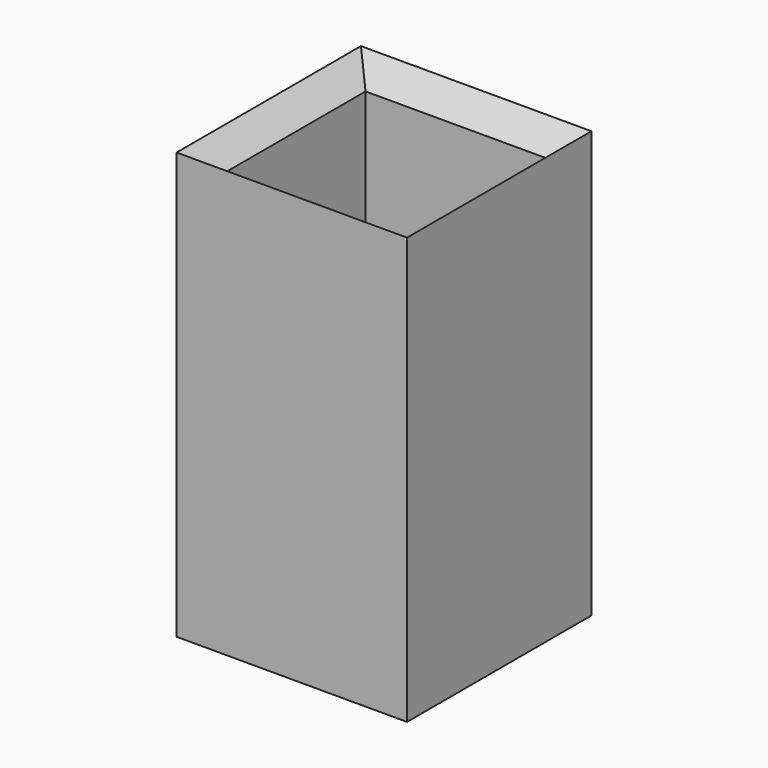
from build123d import *

# Parameters (mm, degrees)
F0_W         = 25.4
F0_H         = 25.4
F0_W_2       = 20.32
F0_H_2       = 20.32
F1_DEPTH     = 50.8
F2_T1_DEPTH  = 20.32
F2_T3_DEPTH  = 20.32
F2_T9_DEPTH  = 36.6501869736
F2_T15_DEPTH = 36.6501869736
F2_T24_DEPTH = 36.6501869736
F2_T30_DEPTH = 36.6501869736
F2_T39_DEPTH = 36.6501869736
F2_T45_DEPTH = 36.6501869736
F2_T54_DEPTH = 36.6501869736
F2_T60_DEPTH = 36.6501869736


# Not quite as in the source:
# - a fillet or chamfer that OpenCascade refuses, or shapes differently, is made with other operations: its cross-section is extruded or revolved along the edge and cut away or added


with BuildPart() as f1:
    # F0 (on Top) → F1 (new body)
    with BuildSketch(Plane.XY):
        Rectangle(F0_W, F0_H)
        Rectangle(F0_W_2, F0_H_2, mode=Mode.SUBTRACT)
    extrude(amount=F1_DEPTH)

    # F2: chamfer of 6.35 on 4 edges, made by hand

    # F2_s2 → F2_t1 (cut)
    with BuildSketch(Plane.XZ.offset(-10.16)):
        Polygon((-10.16, 44.45), (-16.51, 50.8), (-10.16, 50.8), align=None)
        Polygon((10.16, 44.45), (16.51, 50.8), (10.16, 50.8), align=None)
    extrude(amount=F2_T1_DEPTH, mode=Mode.SUBTRACT)

    # F2_s4 → F2_t3 (cut)
    with BuildSketch(Plane.YZ.offset(-10.16)):
        Polygon((-10.16, 44.45), (-16.51, 50.8), (-10.16, 50.8), align=None)
        Polygon((10.16, 44.45), (16.51, 50.8), (10.16, 50.8), align=None)
    extrude(amount=F2_T3_DEPTH, mode=Mode.SUBTRACT)


with BuildPart() as f2_tool7:
    # F2_s8 → F2_t9 (new body)
    with BuildSketch(Plane.YZ.offset(10.16)):
        Polygon((-10.16, 44.45), (-16.51, 50.8), (-10.16, 50.8), align=None)
    extrude(amount=-F2_T9_DEPTH)

    split(bisect_by=Plane.XZ.offset(12.7), keep=Keep.BOTTOM)

    split(bisect_by=Plane.YZ.offset(-12.7), keep=Keep.TOP)

    split(bisect_by=Plane.YZ.offset(-10.16), keep=Keep.BOTTOM)


with BuildPart() as f2_tool13:
    # F2_s14 → F2_t15 (new body)
    with BuildSketch(Plane.XZ.offset(26.4901869736)):
        Polygon((-10.16, 44.45), (-16.51, 50.8), (-10.16, 50.8), align=None)
    extrude(amount=-F2_T15_DEPTH)

    split(bisect_by=Plane.XZ.offset(12.7), keep=Keep.BOTTOM)

    split(bisect_by=Plane.YZ.offset(-12.7), keep=Keep.TOP)

    split(bisect_by=Plane.XZ.offset(10.16), keep=Keep.TOP)


with BuildPart() as f2_tool7_1:
    add(f2_tool7.part)

    # F2_t19: intersect F2_tool13
    add(f2_tool13.part, mode=Mode.INTERSECT)


with BuildPart() as f1_1:
    add(f1.part)

    # F2_t5: cut F2_tool7
    add(f2_tool7_1.part, mode=Mode.SUBTRACT)


with BuildPart() as f2_tool22:
    # F2_s23 → F2_t24 (new body)
    with BuildSketch(Plane.YZ.offset(-26.4901869736)):
        Polygon((10.16, 44.45), (16.51, 50.8), (10.16, 50.8), align=None)
    extrude(amount=F2_T24_DEPTH)

    split(bisect_by=Plane.XZ.offset(-12.7), keep=Keep.TOP)

    split(bisect_by=Plane.YZ.offset(-12.7), keep=Keep.TOP)

    split(bisect_by=Plane.YZ.offset(-10.16), keep=Keep.BOTTOM)


with BuildPart() as f2_tool28:
    # F2_s29 → F2_t30 (new body)
    with BuildSketch(Plane.XZ.offset(10.16)):
        Polygon((-10.16, 44.45), (-16.51, 50.8), (-10.16, 50.8), align=None)
    extrude(amount=-F2_T30_DEPTH)

    split(bisect_by=Plane.XZ.offset(-12.7), keep=Keep.TOP)

    split(bisect_by=Plane.YZ.offset(-12.7), keep=Keep.TOP)

    split(bisect_by=Plane.XZ.offset(-10.16), keep=Keep.BOTTOM)


with BuildPart() as f2_tool22_1:
    add(f2_tool22.part)

    # F2_t34: intersect F2_tool28
    add(f2_tool28.part, mode=Mode.INTERSECT)


with BuildPart() as f1_2:
    add(f1_1.part)

    # F2_t20: cut F2_tool22
    add(f2_tool22_1.part, mode=Mode.SUBTRACT)


with BuildPart() as f2_tool37:
    # F2_s38 → F2_t39 (new body)
    with BuildSketch(Plane.YZ.offset(-10.16)):
        Polygon((10.16, 44.45), (16.51, 50.8), (10.16, 50.8), align=None)
    extrude(amount=F2_T39_DEPTH)

    split(bisect_by=Plane.YZ.offset(12.7), keep=Keep.BOTTOM)

    split(bisect_by=Plane.XZ.offset(-12.7), keep=Keep.TOP)

    split(bisect_by=Plane.YZ.offset(10.16), keep=Keep.TOP)


with BuildPart() as f2_tool43:
    # F2_s44 → F2_t45 (new body)
    with BuildSketch(Plane.XZ.offset(-26.4901869736)):
        Polygon((10.16, 44.45), (16.51, 50.8), (10.16, 50.8), align=None)
    extrude(amount=F2_T45_DEPTH)

    split(bisect_by=Plane.YZ.offset(12.7), keep=Keep.BOTTOM)

    split(bisect_by=Plane.XZ.offset(-12.7), keep=Keep.TOP)

    split(bisect_by=Plane.XZ.offset(-10.16), keep=Keep.BOTTOM)


with BuildPart() as f2_tool37_1:
    add(f2_tool37.part)

    # F2_t49: intersect F2_tool43
    add(f2_tool43.part, mode=Mode.INTERSECT)


with BuildPart() as f1_3:
    add(f1_2.part)

    # F2_t35: cut F2_tool37
    add(f2_tool37_1.part, mode=Mode.SUBTRACT)


with BuildPart() as f2_tool52:
    # F2_s53 → F2_t54 (new body)
    with BuildSketch(Plane.XZ.offset(-10.16)):
        Polygon((10.16, 44.45), (16.51, 50.8), (10.16, 50.8), align=None)
    extrude(amount=F2_T54_DEPTH)

    split(bisect_by=Plane.XZ.offset(12.7), keep=Keep.BOTTOM)

    split(bisect_by=Plane.YZ.offset(12.7), keep=Keep.BOTTOM)

    split(bisect_by=Plane.XZ.offset(10.16), keep=Keep.TOP)


with BuildPart() as f2_tool58:
    # F2_s59 → F2_t60 (new body)
    with BuildSketch(Plane.YZ.offset(26.4901869736)):
        Polygon((-10.16, 44.45), (-16.51, 50.8), (-10.16, 50.8), align=None)
    extrude(amount=-F2_T60_DEPTH)

    split(bisect_by=Plane.XZ.offset(12.7), keep=Keep.BOTTOM)

    split(bisect_by=Plane.YZ.offset(12.7), keep=Keep.BOTTOM)

    split(bisect_by=Plane.YZ.offset(10.16), keep=Keep.TOP)


with BuildPart() as f2_tool52_1:
    add(f2_tool52.part)

    # F2_t64: intersect F2_tool58
    add(f2_tool58.part, mode=Mode.INTERSECT)


with BuildPart() as f1_4:
    add(f1_3.part)

    # F2_t50: cut F2_tool52
    add(f2_tool52_1.part, mode=Mode.SUBTRACT)


solid = f1_4.part
